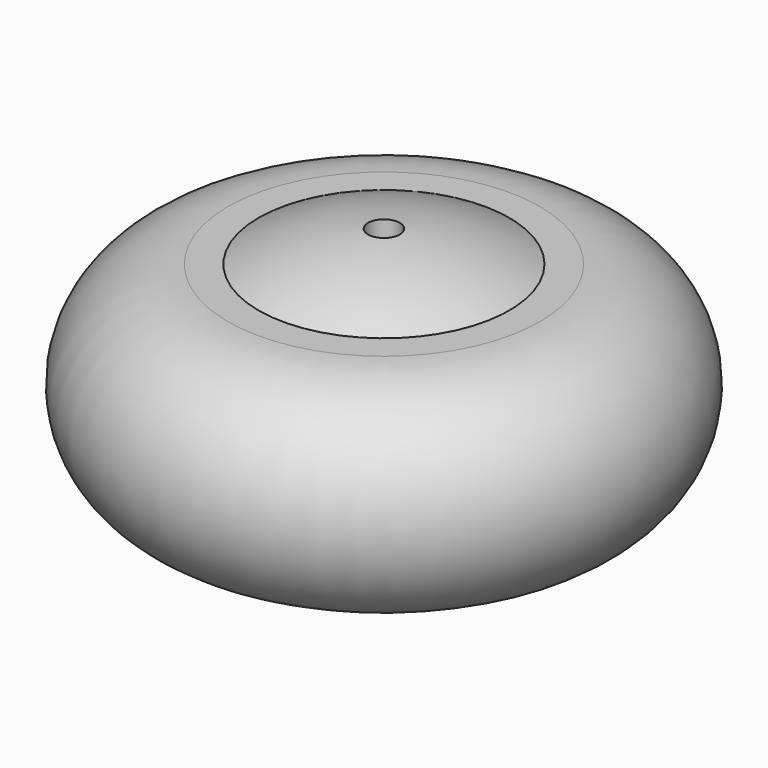
from build123d import *

# Parameters (mm, degrees)
F2_R          = 1.5
F3_DEPTH      = 12.9869215285
F3_DEPTH_BACK = 12.9989252025


with BuildPart() as f1:
    # F0 (on Front) → F1 (revolve)
    with BuildSketch(Plane.XZ):
        with BuildLine():
            Line((-14.3907028701, -9.9814205907), (-11.8812240268, -9.9822056607))
            ThreePointArc((-11.8812240268, -9.9822056607), (-6.127515675, -12.2233626404), (0, -12.9859215285))
            Line((0, -12.9859215285), (0, 12.9979252025))
            ThreePointArc((0, 12.9979252025), (-6.1242831271, 12.2361833119), (-11.8753564136, 9.9973776968))
            Line((-11.8753564136, 9.9973776968), (-14.765259022, 9.997244454))
            ThreePointArc((-14.765259022, 9.997244454), (-24.9909553574, 0.425218823), (-15.6155422227, -9.9810374096))
            Line((-15.6155422227, -9.9810374096), (-14.3907028701, -9.9814205907))
        make_face()
        with BuildLine():
            ThreePointArc((-15.6155422227, -9.9810374096), (-15.0031284186, -9.9999995106), (-14.3907028701, -9.9814205907))
            Line((-14.3907028701, -9.9814205907), (-15.6155422227, -9.9810374096))
        make_face()
    revolve(axis=Axis((0, 0, 0.006001837), (0, 0, -1)))

    # F2 (on Top) → F3 (cut, two sides)
    with BuildSketch(Plane.XY) as f3_sk:
        Circle(F2_R)
    extrude(amount=-F3_DEPTH, mode=Mode.SUBTRACT)
    extrude(f3_sk.sketch, amount=F3_DEPTH_BACK, mode=Mode.SUBTRACT)


solid = f1.part
